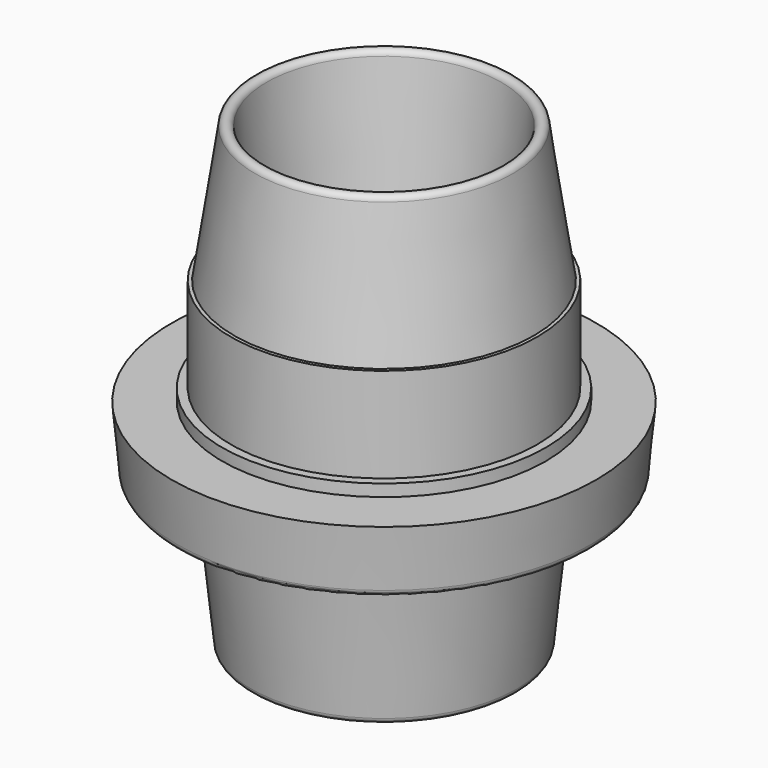
from build123d import *

# Parameters (mm, degrees)
F3_START = -10
F2_R     = 3
F3_DEPTH = 20


with BuildPart() as f1:
    # F0 (on Front) → F1 (revolve)
    with BuildSketch(Plane.XZ):
        with BuildLine():
            Line((62.1, 0), (47.35, 0))
            Line((47.35, 0), (47.35, 3.5))
            Line((47.35, 3.5), (44.85, 3.5))
            Line((44.85, 3.5), (44.85, 31.2))
            Line((44.85, 31.2), (43.85, 31.2))
            Line((43.85, 31.2), (37.8303318608, 71.0116326655))
            ThreePointArc((37.8303318608, 71.0116326655), (36.1, 72.5), (34.3696681392, 71.0116326655))
            Line((34.3696681392, 71.0116326655), (27, 0))
            Line((27, 0), (35.3775171312, -61.4864782954))
            ThreePointArc((35.3775171312, -61.4864782954), (37.1394995022, -63), (38.8521475937, -61.4308708337))
            Line((38.8521475937, -61.4308708337), (43.1, -20.5))
            Line((43.1, -20.5), (58.7000275247, -19))
            ThreePointArc((58.7000275247, -19), (59.9249879423, -18.4212207992), (60.5, -17.194487527))
            Line((60.5, -17.194487527), (62.1, 0))
        make_face()
    revolve(axis=Axis((0, 0, -1.9075102699), (0, 0, -1)))

    # F2 (on Top) → F3 (cut)
    with BuildSketch(Plane.XY.offset(F3_START)):
        with Locations((0, 55)):
            Circle(F2_R)
        with Locations((-55, 0)):
            Circle(F2_R)
        with Locations((55, 0)):
            Circle(F2_R)
        with Locations((0, -55)):
            Circle(F2_R)
    extrude(amount=-F3_DEPTH, mode=Mode.SUBTRACT)


solid = f1.part
